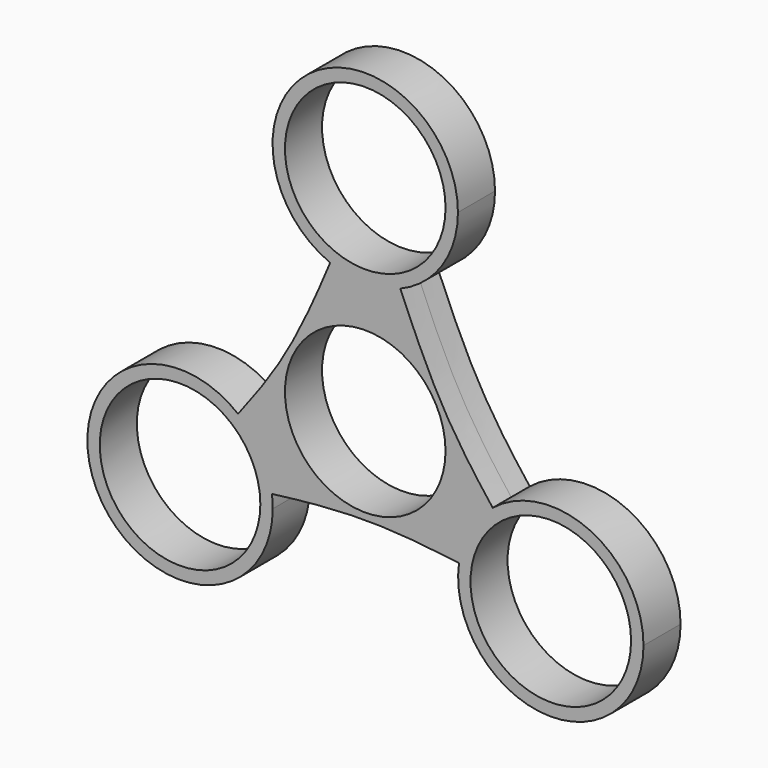
from build123d import *

# Parameters (mm, degrees)
F0_R     = 11
F2_DEPTH = 3.175
F1_R     = 11
F3_DEPTH = 12.7


with BuildPart() as f2:
    # F0 (on Front) → F2 (new body, symmetric)
    with BuildSketch(Plane.XZ):
        with BuildLine():
            ThreePointArc((4.802556, 33.259754), (10.542354, 37.935107), (12.7, 45.016686))
            ThreePointArc((12.7, 45.016686), (-7.082347, 55.558525), (-4.800845, 33.259055))
            add(Edge.make_bspline(
                [(-4.800845, 33.259055), (-3.444226, 36.497411), (-1.896808, 40.324942), (0, 45.016686)],
                knots=[41.442702, 41.442702, 41.442702, 41.442702, 50.8, 50.8, 50.8, 50.8], degree=3))
            add(Edge.make_bspline(
                [(0, 45.016686), (1.898389, 40.32204), (3.445587, 36.495875), (4.802556, 33.259754)],
                knots=[0, 0, 0, 0, 9.397698, 9.397698, 9.397698, 9.397698], degree=3))
        make_face()
        with BuildLine():
            add(Edge.make_bspline(
                [(-4.800845, 33.259055), (-3.444226, 36.497411), (-1.896808, 40.324942), (0, 45.016686)],
                knots=[41.442702, 41.442702, 41.442702, 41.442702, 50.8, 50.8, 50.8, 50.8], degree=3))
            ThreePointArc((-4.800845, 33.259055), (0.000924, 32.316686), (4.802556, 33.259754))
            add(Edge.make_bspline(
                [(0, 45.016686), (1.898389, 40.32204), (3.445587, 36.495875), (4.802556, 33.259754)],
                knots=[0, 0, 0, 0, 9.397698, 9.397698, 9.397698, 9.397698], degree=3))
        make_face()
        with BuildLine():
            ThreePointArc((4.802556, 33.259754), (0.000924, 32.316686), (-4.800845, 33.259055))
            add(Edge.make_bspline(
                [(-17.426131, 10.912862), (-11.603577, 18.432847), (-9.209884, 22.73433), (-4.800845, 33.259055)],
                knots=[11.031287, 11.031287, 11.031287, 11.031287, 41.442702, 41.442702, 41.442702, 41.442702], degree=3))
            ThreePointArc((-17.426131, 10.912862), (-14.333876, 7.283122), (-12.79817, 2.76885))
            add(Edge.make_bspline(
                [(12.844689, 2.780403), (2.448726, 4.09479), (-2.42729, 4.092977), (-12.79817, 2.76885)],
                knots=[10.130243, 10.130243, 10.130243, 10.130243, 40.649094, 40.649094, 40.649094, 40.649094], degree=3))
            ThreePointArc((12.844689, 2.780403), (14.375082, 7.297871), (17.463961, 10.932213))
            add(Edge.make_bspline(
                [(4.802556, 33.259754), (9.196093, 22.781984), (11.595455, 18.48968), (17.463961, 10.932213)],
                knots=[9.397698, 9.397698, 9.397698, 9.397698, 39.82515, 39.82515, 39.82515, 39.82515], degree=3))
        make_face()
        with Locations((0, 15.677886)):
            Circle(F0_R, mode=Mode.SUBTRACT)
        with BuildLine():
            add(Edge.make_bspline(
                [(-25.375577, 1.008504), (-22.101378, 5.033857), (-19.538175, 8.185099), (-17.426131, 10.912862)],
                knots=[0, 0, 0, 0, 11.031287, 11.031287, 11.031287, 11.031287], degree=3))
            ThreePointArc((-17.426131, 10.912862), (-36.826516, -4.483855), (-12.675577, 1.008504))
            ThreePointArc((-12.675577, 1.008504), (-12.706262, 1.890809), (-12.79817, 2.76885))
            add(Edge.make_bspline(
                [(-12.79817, 2.76885), (-16.247638, 2.328431), (-20.305004, 1.741724), (-25.375577, 1.008504)],
                knots=[40.649094, 40.649094, 40.649094, 40.649094, 50.8, 50.8, 50.8, 50.8], degree=3))
        make_face()
        with BuildLine():
            ThreePointArc((-12.79817, 2.76885), (-14.333876, 7.283122), (-17.426131, 10.912862))
            add(Edge.make_bspline(
                [(-25.375577, 1.008504), (-22.101378, 5.033857), (-19.538175, 8.185099), (-17.426131, 10.912862)],
                knots=[0, 0, 0, 0, 11.031287, 11.031287, 11.031287, 11.031287], degree=3))
            add(Edge.make_bspline(
                [(-12.79817, 2.76885), (-16.247638, 2.328431), (-20.305004, 1.741724), (-25.375577, 1.008504)],
                knots=[40.649094, 40.649094, 40.649094, 40.649094, 50.8, 50.8, 50.8, 50.8], degree=3))
        make_face()
        with BuildLine():
            add(Edge.make_bspline(
                [(17.463961, 10.932213), (19.580667, 8.206318), (22.148698, 5.055635), (25.424415, 1.036701)],
                knots=[39.82515, 39.82515, 39.82515, 39.82515, 50.8, 50.8, 50.8, 50.8], degree=3))
            ThreePointArc((17.463961, 10.932213), (14.375082, 7.297871), (12.844689, 2.780403))
            add(Edge.make_bspline(
                [(25.424415, 1.036701), (20.354425, 1.762805), (16.295462, 2.344113), (12.844689, 2.780403)],
                knots=[0, 0, 0, 0, 10.130243, 10.130243, 10.130243, 10.130243], degree=3))
        make_face()
        with BuildLine():
            ThreePointArc((38.124415, 1.036701), (30.910408, 12.49069), (17.463961, 10.932213))
            add(Edge.make_bspline(
                [(17.463961, 10.932213), (19.580667, 8.206318), (22.148698, 5.055635), (25.424415, 1.036701)],
                knots=[39.82515, 39.82515, 39.82515, 39.82515, 50.8, 50.8, 50.8, 50.8], degree=3))
            add(Edge.make_bspline(
                [(25.424415, 1.036701), (20.354425, 1.762805), (16.295462, 2.344113), (12.844689, 2.780403)],
                knots=[0, 0, 0, 0, 10.130243, 10.130243, 10.130243, 10.130243], degree=3))
            ThreePointArc((12.844689, 2.780403), (24.550492, -11.633195), (38.124415, 1.036701))
        make_face()
    extrude(amount=F2_DEPTH, both=True)

    # F1 (on Front) → F3 (cut, symmetric)
    with BuildSketch(Plane.XZ):
        with Locations((0, 45.008477)):
            Circle(F1_R)
        with Locations((25.423015, 1.04877)):
            Circle(F1_R)
        with Locations((-25.373796, 1.009265)):
            Circle(F1_R)
    extrude(amount=F3_DEPTH, both=True, mode=Mode.SUBTRACT)


solid = f2.part
